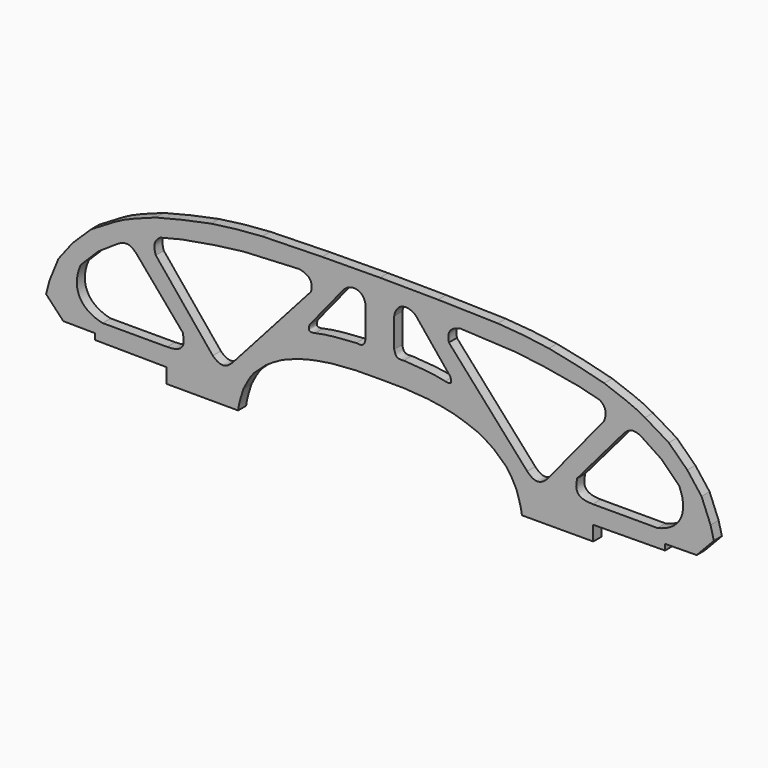
from build123d import *

# Parameters (mm, degrees)
F1_DEPTH = 3


# Not quite as in the source:
# - ends of sketch curves that miss each other by under 0.0002 mm in the source are joined


with BuildPart() as f1:
    # F0 (on Front) → F1 (new body)
    with BuildSketch(Plane.XZ):
        with BuildLine():
            Line((17.292411, 22.4886673102), (0, 22.6303943102))
            Line((0, 22.6303943102), (0, -4.0168806898))
            Line((0, -4.0168806898), (7.228795, -4.0700556898))
            Line((7.228795, -4.0700556898), (14.3159177513, -4.5838576898))
            add(Edge.make_bspline(
                [(22.1116757513, -6.0012756898), (19.5885557513, -5.3778676898), (16.9721657513, -4.9410076898), (14.3159177513, -4.5838576898)],
                knots=[0, 0, 0, 0, 1, 1, 1, 1], degree=3))
            add(Edge.make_bspline(
                [(29.0569877513, -8.4108676898), (26.8431947513, -7.4725876898), (24.5259177513, -6.6722926898), (22.1116757513, -6.0012756898)],
                knots=[0, 0, 0, 0, 1, 1, 1, 1], degree=3))
            add(Edge.make_bspline(
                [(34.0179267513, -11.3874226898), (32.6589677513, -10.4530956898), (31.2598277513, -9.5108856898), (29.0569877513, -8.4108676898)],
                knots=[0, 0, 0, 0, 1, 1, 1, 1], degree=3))
            Line((34.0179267513, -11.3874226898), (37.7031947513, -14.7537826898))
            add(Edge.make_bspline(
                [(40.7151917513, -19.7501556898), (39.9025247513, -18.1165876898), (39.0710207513, -16.4798776898), (37.7031947513, -14.7537826898)],
                knots=[0, 0, 0, 0, 1, 1, 1, 1], degree=3))
            add(Edge.make_bspline(
                [(42.3452147513, -26.0221956898), (42.1316587513, -23.8985406898), (41.3798467513, -21.8287056898), (40.7151917513, -19.7501556898)],
                knots=[0, 0, 0, 0, 1, 1, 1, 1], degree=3))
            Line((42.3452147513, -26.0221956898), (63.6418097513, -25.9867956898))
            Line((63.6418097513, -25.9867956898), (63.6418097513, -21.5928156898))
            Line((63.6418097513, -21.5928156898), (85.0611677513, -21.3930906898))
            Line((85.0611677513, -21.3930906898), (85.0783427513, -19.6170306898))
            Line((85.0783427513, -19.6170306898), (94.5155407513, -19.5168076898))
            Line((94.5155407513, -19.5168076898), (99.6440177513, -14.0805456898))
            Line((99.6440177513, -14.0805456898), (98.6518277513, -10.2535206898))
            Line((98.6518277513, -10.2535206898), (95.9587507513, -3.5916906898))
            Line((95.9587507513, -3.5916906898), (91.7065207513, 1.9361993102))
            Line((91.7065207513, 1.9361993102), (86.1786157513, 7.3223693102))
            Line((86.1786157513, 7.3223693102), (79.0915657513, 11.5746073102))
            add(Edge.make_bspline(
                [(66.9018327513, 16.6772693102), (71.1556647513, 15.1125143102), (75.6872037513, 13.6136843102), (79.0915657513, 11.5746073102)],
                knots=[0, 0, 0, 0, 1, 1, 1, 1], degree=3))
            add(Edge.make_bspline(
                [(50.3932967513, 20.4463193102), (56.1680017513, 19.3841543102), (61.5919797513, 18.0714743102), (66.9018327513, 16.6772693102)],
                knots=[0, 0, 0, 0, 1, 1, 1, 1], degree=3))
            add(Edge.make_bspline(
                [(35.1518327513, 22.0634393102), (40.4118917513, 21.7338963102), (45.5332607513, 21.2425493102), (50.3932967513, 20.4463193102)],
                knots=[0, 0, 0, 0, 1, 1, 1, 1], degree=3))
            Line((35.1518327513, 22.0634393102), (17.292411, 22.4886673102))
        make_face()
        with BuildLine():
            add(Edge.make_bspline(
                [(72.7132127513, 5.3379973102), (73.9598487513, 6.5501393102), (75.1615877513, 7.8382423102), (78.0993757513, 6.1884373102)],
                knots=[0, 0, 0, 0, 1, 1, 1, 1], degree=3))
            Line((78.0993757513, 6.1884373102), (84.0525007513, 2.2196843102))
            Line((84.0525007513, 2.2196843102), (89.2969207513, -3.0247356898))
            add(Edge.make_bspline(
                [(89.2969207513, -3.0247356898), (91.9198887513, -8.8158756898), (90.2818957513, -14.5270806898), (82.7768327513, -16.2066456898)],
                knots=[0, 0, 0, 0, 1, 1, 1, 1], degree=3))
            Line((82.7768327513, -16.2066456898), (63.5000457513, -16.2066456898))
            add(Edge.make_bspline(
                [(63.5000457513, -16.2066456898), (57.1380727513, -16.1648706898), (58.7067867513, -12.4673406898), (58.8225907513, -10.9622406898)],
                knots=[0, 0, 0, 0, 1, 1, 1, 1], degree=3))
            Line((58.8225907513, -10.9622406898), (72.7132127513, 5.3379973102))
        make_face(mode=Mode.SUBTRACT)
        with BuildLine():
            add(Edge.make_bspline(
                [(4.2522797513, 13.9133163102), (5.0251887513, 18.5193293102), (9.4633147513, 17.9503943102), (11.1621567513, 15.5787743102)],
                knots=[0, 0, 0, 0, 1, 1, 1, 1], degree=3))
            Line((11.1621567513, 15.5787743102), (20.9422897513, 3.5307823102))
            add(Edge.make_bspline(
                [(20.9422897513, 3.5307823102), (21.3510167513, 2.4878923102), (21.7530967513, 1.2352573102), (19.4311007513, 1.7529523102)],
                knots=[0, 0, 0, 0, 1, 1, 1, 1], degree=3))
            add(Edge.make_bspline(
                [(19.4311007513, 1.7529523102), (15.4182557513, 2.7136493102), (11.2374477513, 2.8345273102), (7.0996287513, 3.1703543102)],
                knots=[0, 0, 0, 0, 1, 1, 1, 1], degree=3))
            add(Edge.make_bspline(
                [(7.0996287513, 3.1703543102), (4.4484227513, 2.8037243102), (4.6391687513, 4.0357343102), (4.2522797513, 5.1962473102)],
                knots=[0, 0, 0, 0, 1, 1, 1, 1], degree=3))
            Line((4.2522797513, 5.1962473102), (4.2522797513, 13.9133163102))
        make_face(mode=Mode.SUBTRACT)
        with BuildLine():
            add(Edge.make_bspline(
                [(20.5525017513, 12.2833043102), (20.0676617513, 14.6816013102), (20.5440417513, 16.3586093102), (24.0960287513, 17.0670743102)],
                knots=[0, 0, 0, 0, 1, 1, 1, 1], degree=3))
            Line((24.0960287513, 17.0670743102), (40.6797337513, 16.2520573102))
            Line((40.6797337513, 16.2520573102), (49.4676807513, 15.1181243102))
            Line((49.4676807513, 15.1181243102), (59.2478147513, 13.4172363102))
            Line((59.2478147513, 13.4172363102), (65.4844207513, 11.8580763102))
            add(Edge.make_bspline(
                [(65.4844207513, 11.8580763102), (67.5337397513, 10.6827963102), (67.6491757513, 8.8628913102), (66.9018317513, 6.7553913102)],
                knots=[0, 0, 0, 0, 1, 1, 1, 1], degree=3))
            Line((66.9018317513, 6.7553913102), (49.8929027513, -14.0805456898))
            add(Edge.make_bspline(
                [(49.8929027513, -14.0805456898), (47.2968437513, -16.6023676898), (45.5455047513, -15.5763756898), (43.9397777513, -13.9388026898)],
                knots=[0, 0, 0, 0, 1, 1, 1, 1], degree=3))
            Line((43.9397777513, -13.9388026898), (20.5525017513, 12.2833043102))
        make_face(mode=Mode.SUBTRACT)
    extrude(amount=F1_DEPTH)

    # F2: F1 across plane


with BuildPart() as f1_1:
    add(f1.part)
    add(f1.part.mirror(Plane.YZ))


solid = f1_1.part
